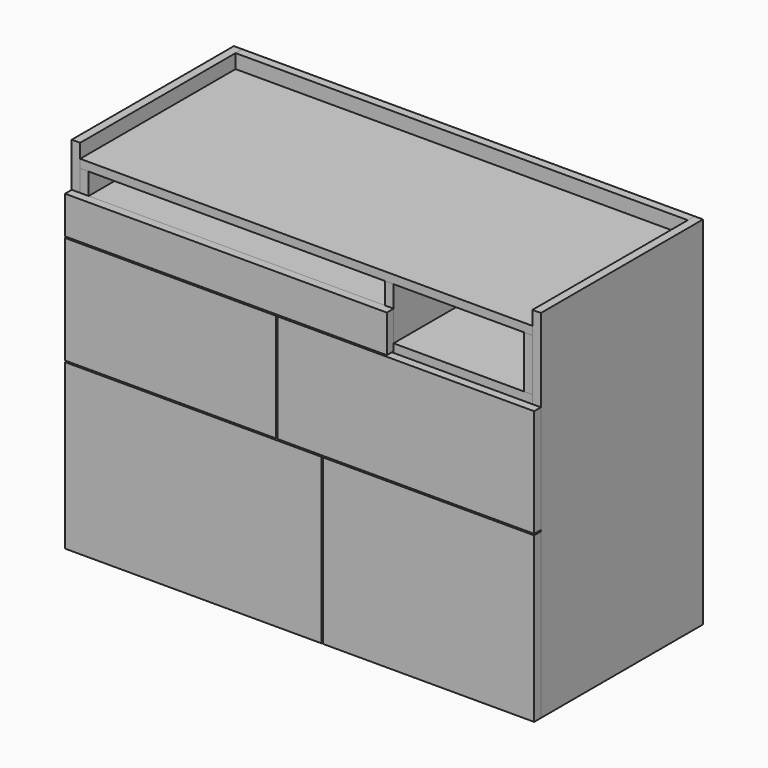
from build123d import *

# Parameters (mm, degrees)
F0_W           = 18
F0_H           = 414
F0_H_2         = 18
F1_DEPTH       = 760
F0_W_2         = 964
F2_DEPTH       = 760
F3_DEPTH       = 20
F3_DEPTH_BACK  = 10
F4_W           = 650
F4_H           = 300
F4_H_2         = 114
F5_DEPTH       = 18
F7_W           = 432
F7_H           = 230
F7_W_2         = 18
F8_DEPTH       = 18
F7_W_3         = 300
F7_W_4         = 244
F7_W_5         = 3
F7_W_6         = 450
F7_H_2         = 350
F7_W_7         = 226
F7_W_8         = 650
F7_H_3         = 80
F10_DEPTH      = 414
F9_W           = 278
F9_H           = 18
F9_W_2         = 18
F9_W_3         = 632
F9_H_2         = 15
F9_H_3         = 3
F11_DEPTH      = 414
F9_H_4         = 7.5
F9_H_5         = 159.5
F9_H_6         = 291.25041
F9_H_7         = 10
F9_H_8         = 111
F9_H_9         = 46
F9_H_10        = 65
F12_W          = 928
F12_H          = 111
F13_DEPTH      = 12
F9_W_4         = 15
F9_W_5         = 358.5
F14_DEPTH      = 400
F9_W_6         = 455.5
F9_H_11        = 67
F9_H_12        = 240
F9_W_7         = 358.8239558978
F9_H_13        = 51.25041
F9_W_8         = 455.1760441022
F9_H_14        = 40
F15_W          = 455.5
F15_H          = 15
F15_W_2        = 15
F16_DEPTH      = 40
F16_DEPTH_BACK = 10
F18_W          = 12
F18_H          = 31
F18_H_2        = 10
F18_W_2        = 578
F19_DEPTH      = 380
F20_W          = 578
F20_H          = 12
F21_DEPTH      = 31
F22_DEPTH      = 18
F18_W_3        = 15
F18_H_3        = 12
F23_DEPTH      = 380
F24_W          = 632
F24_H          = 12
F25_DEPTH      = 46


# Not quite as in the source:
# - a feature names something its author has since deleted; it is built from what else it names


with BuildPart() as f1:
    # F0 (on Top) → F1 (new body)
    with BuildSketch(Plane.XY):
        with Locations((9, 207)):
            Rectangle(F0_W, F0_H)
        with Locations((9, 423)):
            Rectangle(F0_W, F0_H_2)
    extrude(amount=F1_DEPTH)


with BuildPart() as f1b:
    # F0 (on Top) → F1, piece 2 (new body)
    with BuildSketch(Plane.XY):
        with Locations((991, 207)):
            Rectangle(F0_W, F0_H)
        with Locations((991, 423)):
            Rectangle(F0_W, F0_H_2)
    extrude(amount=F1_DEPTH)


with BuildPart() as f2:
    # F0 (on Top) → F2 (new body, through all)
    with BuildSketch(Plane.XY):
        with Locations((500, 423)):
            Rectangle(F0_W_2, F0_H_2)
    extrude(amount=F2_DEPTH)


with BuildPart() as f3:
    # F0 (on Top) → F3 (new body, two sides)
    with BuildSketch(Plane.XY) as f3_sk:
        with Locations((500, 207)):
            Rectangle(F0_W_2, F0_H)
    extrude(amount=F3_DEPTH)
    extrude(f3_sk.sketch, amount=-F3_DEPTH_BACK)


with BuildPart() as f5:
    # F4 (on face) → F5 (new body)
    with BuildSketch(Plane.XY.offset(760)):
        Polygon((982, 414), (668, 414), (668, 300), (668, 0), (982, 0), align=None)
        with Locations((343, 150)):
            Rectangle(F4_W, F4_H)
        with Locations((343, 357)):
            Rectangle(F4_W, F4_H_2)
    extrude(amount=-F5_DEPTH)


with BuildPart() as f5_1:
    # F6: moved
    add(f5.part.moved(Location((0, 0, -30))))


with BuildPart() as f8:
    # F7 (on face) → F8 (new body)
    with BuildSketch(Plane.XZ):
        with Locations((234, 468)):
            Rectangle(F7_W, F7_H)
        with Locations((9, 468)):
            Rectangle(F7_W_2, F7_H)
    extrude(amount=F8_DEPTH)


with BuildPart() as f8b:
    # F7 (on face) → F8, piece 2 (new body)
    with BuildSketch(Plane.XZ):
        with Locations((603, 468)):
            Rectangle(F7_W_3, F7_H)
        with Locations((878, 468)):
            Rectangle(F7_W_4, F7_H)
        with Locations((754.5, 468)):
            Rectangle(F7_W_5, F7_H)
    extrude(amount=F8_DEPTH)


with BuildPart() as f8c:
    # F7 (on face) → F8, piece 3 (new body)
    with BuildSketch(Plane.XZ):
        with Locations((775, 175)):
            Rectangle(F7_W_6, F7_H_2)
    extrude(amount=F8_DEPTH)


with BuildPart() as f8d:
    # F7 (on face) → F8, piece 4 (new body)
    with BuildSketch(Plane.XZ):
        with Locations((397, 175)):
            Rectangle(F7_W_3, F7_H_2)
        with Locations((131, 175)):
            Rectangle(F7_W_7, F7_H_2)
        with Locations((9, 175)):
            Rectangle(F7_W_2, F7_H_2)
        with Locations((245.5, 175)):
            Rectangle(F7_W_5, F7_H_2)
    extrude(amount=F8_DEPTH)


with BuildPart() as f8e:
    # F7 (on face) → F8, piece 5 (new body)
    with BuildSketch(Plane.XZ):
        with Locations((343, 626)):
            Rectangle(F7_W_8, F7_H_3)
        with Locations((9, 626)):
            Rectangle(F7_W_2, F7_H_3)
    extrude(amount=F8_DEPTH)

    # F22 (add, through all): a face of the model
    f22_faces = [f8e.faces().sort_by_distance(p)[0] for p in [
        (668, -9, 626),
    ]]
    extrude(f22_faces, amount=F22_DEPTH)


with BuildPart() as f10:
    # F9 (on face) → F10 (new body, through all)
    with BuildSketch(Plane(origin=(0, 0, 0), x_dir=(-1, 0, 0), z_dir=(0, 1, 0))):
        Polygon((-18, 365), (-36, 365), (-51, 365), (-442.5, 365), (-460.5, 365), (-964, 365), (-982, 365), (-982, 343.75041), (-964, 343.75041), (-949, 343.75041), (-590.1760441022, 343.75041), (-575.1760441022, 343.75041), (-557.1760441022, 343.75041), (-539.1760441022, 343.75041), (-521.1760441022, 343.75041), (-506.1760441022, 343.75041), (-51, 343.75041), (-36, 343.75041), (-18, 343.75041), align=None)
    extrude(amount=F10_DEPTH)


with BuildPart() as f10b:
    # F9 (on face) → F10, piece 2 (new body, through all)
    with BuildSketch(Plane(origin=(0, 0, 0), x_dir=(-1, 0, 0), z_dir=(0, 1, 0))):
        Polygon((-18, 574), (-18, 583), (-36, 583), (-668, 583), (-686, 583), (-964, 583), (-982, 583), (-982, 574), (-424.5, 574), (-409.5, 574), align=None)
        with Locations((-825, 592)):
            Rectangle(F9_W, F9_H)
        Polygon((-686, 583), (-668, 583), (-668, 586), (-668, 601), (-686, 601), align=None)
        with Locations((-973, 592)):
            Rectangle(F9_W_2, F9_H)
        with Locations((-352, 593.5)):
            Rectangle(F9_W_3, F9_H_2)
        with Locations((-27, 593.5)):
            Rectangle(F9_W_2, F9_H_2)
        with Locations((-27, 584.5)):
            Rectangle(F9_W_2, F9_H_3)
        with Locations((-352, 584.5)):
            Rectangle(F9_W_3, F9_H_3)
    extrude(amount=F10_DEPTH)


with BuildPart() as f11:
    # F9 (on face) → F11 (new body, through all)
    with BuildSketch(Plane(origin=(0, 0, 0), x_dir=(-1, 0, 0), z_dir=(0, 1, 0))):
        Polygon((-686, 712), (-686, 601), (-668, 601), (-668, 666), (-668, 712), align=None)
    extrude(amount=F11_DEPTH)


with BuildPart() as f11b:
    # F9 (on face) → F11, piece 2 (new body, through all)
    with BuildSketch(Plane(origin=(0, 0, 0), x_dir=(-1, 0, 0), z_dir=(0, 1, 0))):
        with Locations((-451.5, 561.25)):
            Rectangle(F9_W_2, F9_H_4)
        with Locations((-451.5, 477.75)):
            Rectangle(F9_W_2, F9_H_5)
        with Locations((-451.5, 390.5)):
            Rectangle(F9_W_2, F9_H_2)
        with Locations((-451.5, 374)):
            Rectangle(F9_W_2, F9_H)
    extrude(amount=F11_DEPTH)


with BuildPart() as f11c:
    # F9 (on face) → F11, piece 3 (new body, through all)
    with BuildSketch(Plane(origin=(0, 0, 0), x_dir=(-1, 0, 0), z_dir=(0, 1, 0))):
        with Locations((-548.1760441022, 340.00041)):
            Rectangle(F9_W_2, F9_H_4)
        with Locations((-548.1760441022, 190.625205)):
            Rectangle(F9_W_2, F9_H_6)
        with Locations((-548.1760441022, 40)):
            Rectangle(F9_W_2, F9_H_7)
        with Locations((-548.1760441022, 27.5)):
            Rectangle(F9_W_2, F9_H_2)
    extrude(amount=F11_DEPTH)


with BuildPart() as f11d:
    # F9 (on face) → F11, piece 4 (new body, through all)
    with BuildSketch(Plane(origin=(0, 0, 0), x_dir=(-1, 0, 0), z_dir=(0, 1, 0))):
        with Locations((-973, 656.5)):
            Rectangle(F9_W_2, F9_H_8)
    extrude(amount=F11_DEPTH)


with BuildPart() as f11e:
    # F9 (on face) → F11, piece 5 (new body, through all)
    with BuildSketch(Plane(origin=(0, 0, 0), x_dir=(-1, 0, 0), z_dir=(0, 1, 0))):
        with Locations((-27, 689)):
            Rectangle(F9_W_2, F9_H_9)
        with Locations((-27, 633.5)):
            Rectangle(F9_W_2, F9_H_10)
    extrude(amount=F11_DEPTH)


with BuildPart() as f13:
    # F12 (on face) → F13 (new body)
    with BuildSketch(Plane.XZ.offset(-414)):
        with Locations((500, 656.5)):
            Rectangle(F12_W, F12_H)
    extrude(amount=F13_DEPTH)


with BuildPart() as f14:
    # F9 (on face) → F14 (new body)
    with BuildSketch(Plane(origin=(0, 0, 0), x_dir=(-1, 0, 0), z_dir=(0, 1, 0))):
        with Locations((-43.5, 477.75)):
            Rectangle(F9_W_4, F9_H_5)
        with Locations((-43.5, 390.5)):
            Rectangle(F9_W_4, F9_H_2)
        with Locations((-230.25, 390.5)):
            Rectangle(F9_W_5, F9_H_2)
        with Locations((-417, 390.5)):
            Rectangle(F9_W_4, F9_H_2)
        with Locations((-417, 477.75)):
            Rectangle(F9_W_4, F9_H_5)
    extrude(amount=F14_DEPTH)


with BuildPart() as f14b:
    # F9 (on face) → F14, piece 2 (new body)
    with BuildSketch(Plane(origin=(0, 0, 0), x_dir=(-1, 0, 0), z_dir=(0, 1, 0))):
        with Locations((-486, 390.5)):
            Rectangle(F9_W_4, F9_H_2)
        with Locations((-721.25, 390.5)):
            Rectangle(F9_W_6, F9_H_2)
        with Locations((-956.5, 390.5)):
            Rectangle(F9_W_4, F9_H_2)
        with Locations((-956.5, 431.5)):
            Rectangle(F9_W_4, F9_H_11)
        with Locations((-486, 431.5)):
            Rectangle(F9_W_4, F9_H_11)
    extrude(amount=F14_DEPTH)


with BuildPart() as f14c:
    # F9 (on face) → F14, piece 3 (new body)
    with BuildSketch(Plane(origin=(0, 0, 0), x_dir=(-1, 0, 0), z_dir=(0, 1, 0))):
        with Locations((-956.5, 165)):
            Rectangle(F9_W_4, F9_H_12)
        with Locations((-956.5, 40)):
            Rectangle(F9_W_4, F9_H_7)
        with Locations((-769.5880220511, 40)):
            Rectangle(F9_W_7, F9_H_7)
        with Locations((-582.6760441022, 40)):
            Rectangle(F9_W_4, F9_H_7)
        with Locations((-582.6760441022, 165)):
            Rectangle(F9_W_4, F9_H_12)
        with Locations((-582.6760441022, 310.625205)):
            Rectangle(F9_W_4, F9_H_13)
        with Locations((-956.5, 310.625205)):
            Rectangle(F9_W_4, F9_H_13)
    extrude(amount=F14_DEPTH)


with BuildPart() as f14d:
    # F9 (on face) → F14, piece 4 (new body)
    with BuildSketch(Plane(origin=(0, 0, 0), x_dir=(-1, 0, 0), z_dir=(0, 1, 0))):
        with Locations((-513.6760441022, 40)):
            Rectangle(F9_W_4, F9_H_7)
        with Locations((-513.6760441022, 165)):
            Rectangle(F9_W_4, F9_H_12)
        with Locations((-278.5880220511, 40)):
            Rectangle(F9_W_8, F9_H_7)
        with Locations((-43.5, 40)):
            Rectangle(F9_W_4, F9_H_7)
        with Locations((-43.5, 165)):
            Rectangle(F9_W_4, F9_H_12)
        with Locations((-513.6760441022, 310.625205)):
            Rectangle(F9_W_4, F9_H_13)
        with Locations((-43.5, 310.625205)):
            Rectangle(F9_W_4, F9_H_13)
    extrude(amount=F14_DEPTH)


with BuildPart() as f14e:
    # F9 (on face) → F14, piece 5 (new body)
    with BuildSketch(Plane(origin=(0, 0, 0), x_dir=(-1, 0, 0), z_dir=(0, 1, 0))):
        with Locations((-486, 505)):
            Rectangle(F9_W_4, F9_H_14)
        with Locations((-486, 480)):
            Rectangle(F9_W_4, F9_H_7)
        Polygon((-575.1760441022, 485), (-949, 485), (-949, 475), (-575.1760441022, 475), (-493.5, 475), (-493.5, 485), align=None)
        with Locations((-956.5, 480)):
            Rectangle(F9_W_4, F9_H_7)
        with Locations((-956.5, 505)):
            Rectangle(F9_W_4, F9_H_14)
    extrude(amount=F14_DEPTH)


with BuildPart() as f16:
    # F15 (on face) → F16 (new body, two sides)
    with BuildSketch(Plane.XY.offset(485)) as f16_sk:
        with Locations((721.25, 7.5)):
            Rectangle(F15_W, F15_H)
        with Locations((486, 7.5)):
            Rectangle(F15_W_2, F15_H)
        with Locations((956.5, 7.5)):
            Rectangle(F15_W_2, F15_H)
    extrude(amount=F16_DEPTH)
    extrude(f16_sk.sketch, amount=-F16_DEPTH_BACK)


with BuildPart() as f14e_1:
    add(f14e.part)

    # F17: cut F16
    add(f16.part, mode=Mode.SUBTRACT)


with BuildPart() as f19:
    # F18 (on face) → F19 (new body)
    with BuildSketch(Plane(origin=(0, 0, 0), x_dir=(-1, 0, 0), z_dir=(0, 1, 0))):
        with Locations((-57, 638.5)):
            Rectangle(F18_W, F18_H)
        with Locations((-57, 618)):
            Rectangle(F18_W, F18_H_2)
        with Locations((-352, 618)):
            Rectangle(F18_W_2, F18_H_2)
        with Locations((-647, 618)):
            Rectangle(F18_W, F18_H_2)
        with Locations((-647, 638.5)):
            Rectangle(F18_W, F18_H)
    extrude(amount=F19_DEPTH)


with BuildPart() as f21:
    # F20 (on face) → F21 (new body, through all)
    with BuildSketch(Plane.XY.offset(623)):
        with Locations((352, 374)):
            Rectangle(F20_W, F20_H)
    extrude(amount=F21_DEPTH)


with BuildPart() as f23:
    # F18 (on face) → F23 (new body, through all)
    with BuildSketch(Plane(origin=(0, 0, 0), x_dir=(-1, 0, 0), z_dir=(0, 1, 0))):
        Polygon((-51, 654), (-51, 666), (-653, 666), (-653, 654), (-641, 654), (-63, 654), align=None)
        with Locations((-660.5, 660)):
            Rectangle(F18_W_3, F18_H_3)
        with Locations((-43.5, 660)):
            Rectangle(F18_W_3, F18_H_3)
    extrude(amount=F23_DEPTH)


with BuildPart() as f25:
    # F24 (on face) → F25 (new body, through all)
    with BuildSketch(Plane.XY.offset(666)):
        with Locations((352, 374)):
            Rectangle(F24_W, F24_H)
    extrude(amount=F25_DEPTH)


solid = Compound([f1.part, f1b.part, f2.part, f3.part, f5_1.part, f8.part, f8b.part, f8c.part, f8d.part, f8e.part, f10.part, f10b.part, f11.part, f11b.part, f11c.part, f11d.part, f11e.part, f13.part, f14.part, f14b.part, f14c.part, f14d.part, f16.part, f14e_1.part, f19.part, f21.part, f23.part, f25.part])
